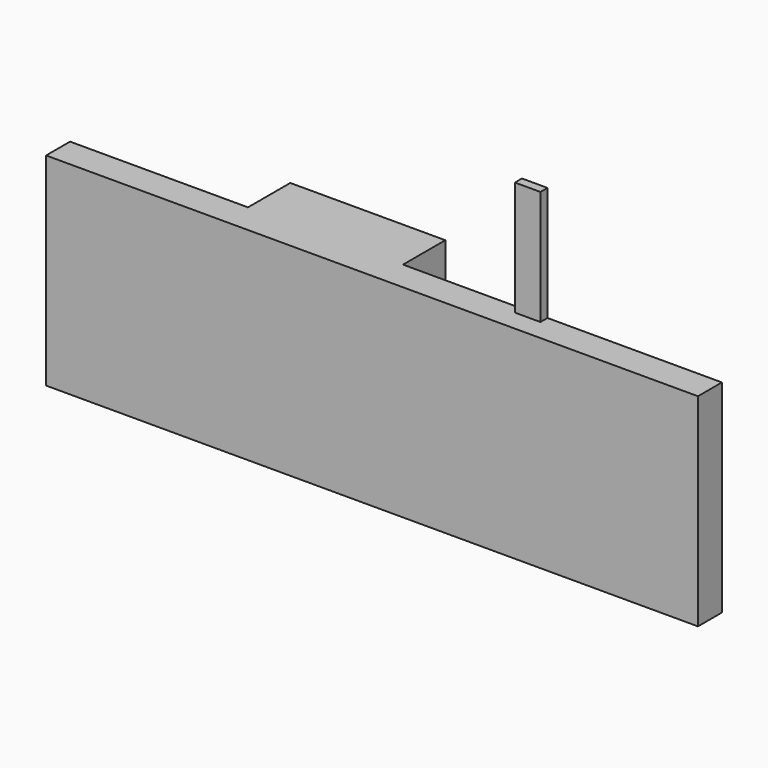
from build123d import *

# Parameters (mm, degrees)
F1_DEPTH = 1150
F0_W     = 145
F0_H     = 50
F2_DEPTH = 1800


# Not quite as in the source:
# - the program builds the solid bodies; features that only make, move or delete a surface that nothing else refers to are left out


with BuildPart() as f1:
    # F0 (on Top) → F1 (new body)
    with BuildSketch(Plane.XY):
        Polygon((-938.0989384058, 395.8452334432), (-1948.0989384058, 395.8452334432), (-1948.0989384058, 225.8452334432), (1751.9010615942, 225.8452334432), (1751.9010615942, 395.8452334432), (761.9010615942, 395.8452334432), (761.9010615942, 345.8452334432), (616.9010615942, 345.8452334432), (616.9010615942, 395.8452334432), (-58.0989384058, 395.8452334432), (-58.0989384058, 695.8452334432), (-938.0989384058, 695.8452334432), align=None)
    extrude(amount=F1_DEPTH)

    # F0 (on Top) → F2 (join)
    with BuildSketch(Plane.XY):
        with Locations((689.4010615942, 370.8452334432)):
            Rectangle(F0_W, F0_H)
    extrude(amount=F2_DEPTH)


solid = f1.part
